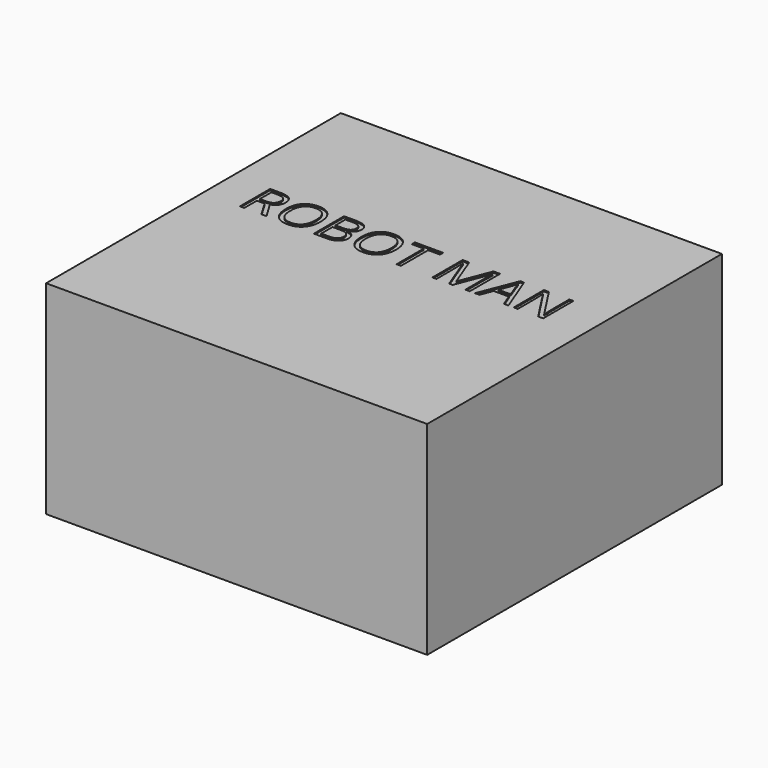
from build123d import *

# Parameters (mm, degrees)
F0_W         = 300
F0_H         = 290
F1_DEPTH     = 160
F2_TEXT_SIZE = 41.6666666667
F3_DEPTH     = 1


# Not quite as in the source:
# - Text() gives the source's letters only with a copy of the font that has no kerning and outlines rounded to 1/6400 em; it was checked with that copy


with BuildPart() as f1:
    # F0 (on Top) → F1 (new body)
    with BuildSketch(Plane.XY):
        Rectangle(F0_W, F0_H)
    extrude(amount=F1_DEPTH)

    # F2 (on face) → F3 (cut)
    with BuildSketch(Plane.XY.offset(160)):
        with Locations((-125, 9.3350558655)):
            Text('ROBOT MAN', F2_TEXT_SIZE, font='Open Sans', text_align=(TextAlign.LEFT, TextAlign.BOTTOM))
    extrude(amount=-F3_DEPTH, mode=Mode.SUBTRACT)


solid = f1.part
